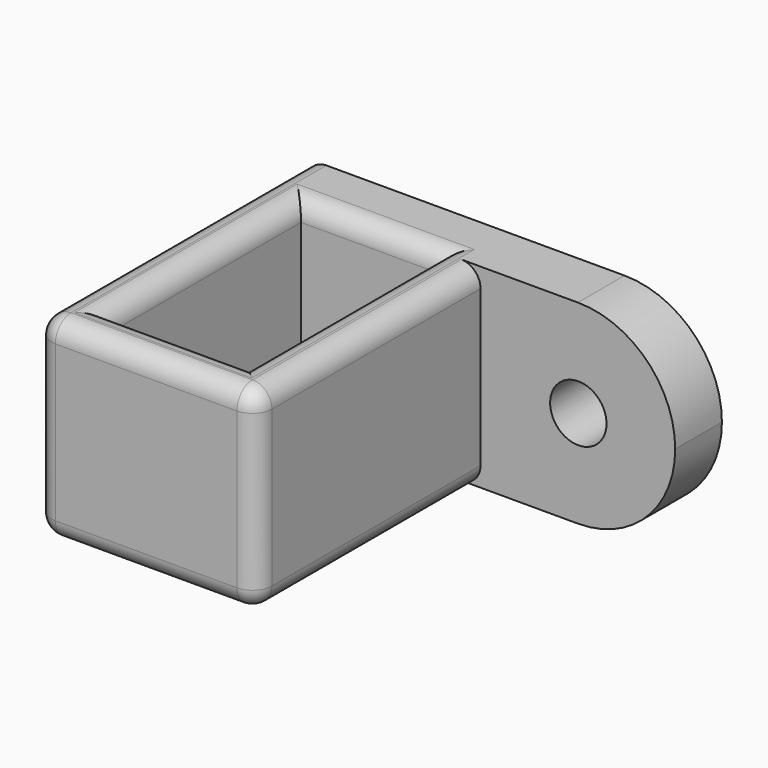
from build123d import *

# Parameters (mm, degrees)
F0_W      = 10
F0_H      = 3
F0_W_2    = 7.1
F0_H_2    = 12.3
F1_DEPTH  = 10
F2_R      = 1.4483503842
F1_FACE_W = 21.323674424
F1_FACE_H = 10
F3_DEPTH  = 15.301
F4_R      = 4.99999
F5_F1_R   = 1
F5_F2_R   = 1
F5_F3_R   = 1
F5_F4_R   = 1
F5_F5_R   = 1
F5_F6_R   = 1
F5_F7_R   = 1
F5_F8_R   = 1
F5_F9_R   = 1
F5_F10_R  = 0.9999
F5_F11_R  = 1
F5_F12_R  = 1
F5_F13_R  = 1


# Not quite as in the source:
# - a fillet or chamfer is up to 0.001 mm smaller than in the source, because OpenCascade refuses the exact size


with BuildPart() as f1:
    # F0 (on Top) → F1 (new body)
    with BuildSketch(Plane.XY):
        with Locations((14.223674424, 13.8)):
            Rectangle(F0_W, F0_H)
        Polygon((-2.1, 12.3), (-2.1, 0), (-2.1, -2.1), (7.1, -2.1), (9.223674424, -2.1), (9.223674424, 12.3), (9.223674424, 15.3), (-2.1, 15.3), (-2.1, 14.4), (-2.0836676853, 12.3), align=None)
        with Locations((3.55, 6.15)):
            Rectangle(F0_W_2, F0_H_2, mode=Mode.SUBTRACT)
    extrude(amount=F1_DEPTH)

    # F2 (on Front) + F1_face (on face) → F3 (cut, through all)
    with BuildSketch(Plane.XZ):
        with Locations((14.2455906607, 4.9976706505)):
            Circle(F2_R)
    with BuildSketch(Plane(origin=(8.561837212, 15.3, 5), x_dir=(-1, 0, 0), z_dir=(0, 1, 0))):
        Rectangle(F1_FACE_W, F1_FACE_H)
    extrude(amount=-F3_DEPTH, dir=(0, -1, 0), mode=Mode.SUBTRACT)

    # F4 (radius 5 in the source; OpenCascade refuses exactly that, so slightly less here)
    f4_edges = [f1.edges().sort_by_distance(p)[0] for p in [
        (19.223674, 13.8, 10),
        (19.223674, 13.8, 0),
    ]]
    fillet(f4_edges, radius=F4_R)

    # F5: fillet of radius 1 on 18 edges, made by hand

    # F5_f1
    f5_f1_edges = [f1.edges().sort_by_distance(p)[0] for p in [
        (9.223674424, 5.1, 0),
    ]]
    fillet(f5_f1_edges, radius=F5_F1_R)

    # F5_f2
    f5_f2_edges = [f1.edges().sort_by_distance(p)[0] for p in [
        (-2.1, 5.1, 0),
    ]]
    fillet(f5_f2_edges, radius=F5_F2_R)

    # F5_f3
    f5_f3_edges = [f1.edges().sort_by_distance(p)[0] for p in [
        (9.223674424, 5.1, 10),
    ]]
    fillet(f5_f3_edges, radius=F5_F3_R)

    # F5_f4
    f5_f4_edges = [f1.edges().sort_by_distance(p)[0] for p in [
        (-2.1, 5.1, 10),
    ]]
    fillet(f5_f4_edges, radius=F5_F4_R)

    # F5_f5
    f5_f5_edges = [f1.edges().sort_by_distance(p)[0] for p in [
        (0, 6.15, 0),
    ]]
    fillet(f5_f5_edges, radius=F5_F5_R)

    # F5_f6
    f5_f6_edges = [f1.edges().sort_by_distance(p)[0] for p in [
        (7.1, 6.15, 0),
    ]]
    fillet(f5_f6_edges, radius=F5_F6_R)

    # F5_f7
    f5_f7_edges = [f1.edges().sort_by_distance(p)[0] for p in [
        (0, 6.15, 10),
    ]]
    fillet(f5_f7_edges, radius=F5_F7_R)

    # F5_f8
    f5_f8_edges = [f1.edges().sort_by_distance(p)[0] for p in [
        (7.1, 6.15, 10),
    ]]
    fillet(f5_f8_edges, radius=F5_F8_R)

    # F5_f9
    f5_f9_edges = [f1.edges().sort_by_distance(p)[0] for p in [
        (3.561837212, -2.1, 0),
    ]]
    fillet(f5_f9_edges, radius=F5_F9_R)

    # F5_f10 (radius 1 in the source; OpenCascade refuses exactly that, so slightly less here)
    f5_f10_edges = [f1.edges().sort_by_distance(p)[0] for p in [
        (3.55, 12.3, 0),
    ]]
    fillet(f5_f10_edges, radius=F5_F10_R)

    # F5_f11
    f5_f11_edges = [f1.edges().sort_by_distance(p)[0] for p in [
        (3.55, 0, 0),
    ]]
    fillet(f5_f11_edges, radius=F5_F11_R)

    # F5_f12
    f5_f12_edges = [f1.edges().sort_by_distance(p)[0] for p in [
        (3.55, 12.3, 10),
    ]]
    fillet(f5_f12_edges, radius=F5_F12_R)

    # F5_f13
    f5_f13_edges = [f1.edges().sort_by_distance(p)[0] for p in [
        (3.55, 0, 10),
    ]]
    fillet(f5_f13_edges, radius=F5_F13_R)


solid = f1.part
